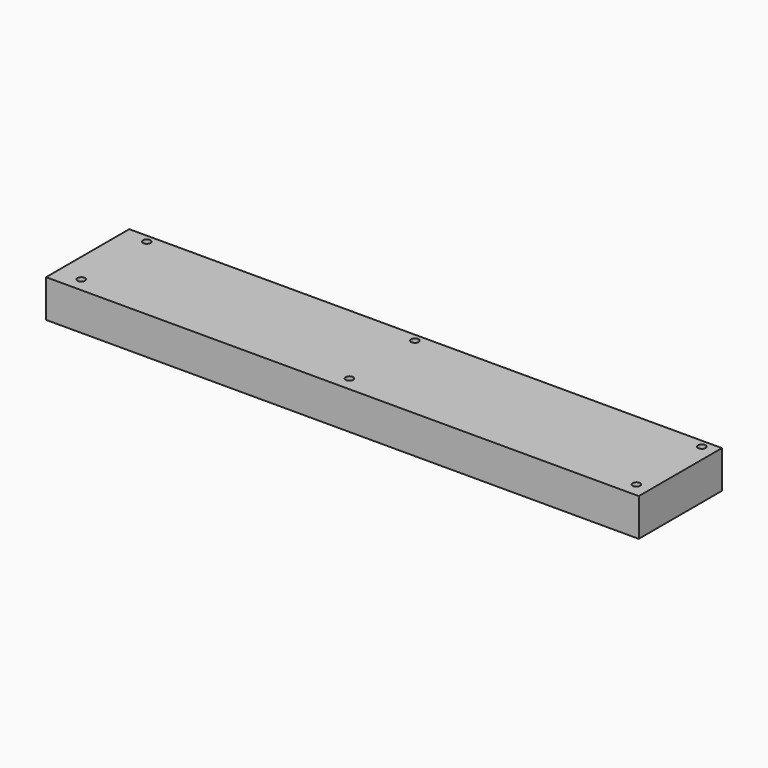
from build123d import *

# Parameters (mm, degrees)
F0_R     = 2.54
F1_DEPTH = 25.4


# Not quite as in the source:
# - ends of sketch curves that miss each other by under 0.0002 mm in the source are joined


with BuildPart() as f1:
    # F0 (on Top) → F1 (new body)
    with BuildSketch(Plane.XY):
        Polygon((1.6850286694, 31.1051446888), (-398.3649713306, 31.1051446888), (-398.3649713306, -39.0623553112), (1.6850335819, -39.0623553112), align=None)
        with Locations((-382.2613713306, -29.4900387525)):
            Circle(F0_R, mode=Mode.SUBTRACT)
        with Locations((-201.2863713306, -29.4900387525)):
            Circle(F0_R, mode=Mode.SUBTRACT)
        with Locations((-7.6113713306, -29.4900387525)):
            Circle(F0_R, mode=Mode.SUBTRACT)
        with Locations((-382.2613713306, 25.7930612475)):
            Circle(F0_R, mode=Mode.SUBTRACT)
        with Locations((-201.2863713306, 25.7930612475)):
            Circle(F0_R, mode=Mode.SUBTRACT)
        with Locations((-7.6113713306, 25.7930612475)):
            Circle(F0_R, mode=Mode.SUBTRACT)
    extrude(amount=F1_DEPTH)


solid = f1.part
